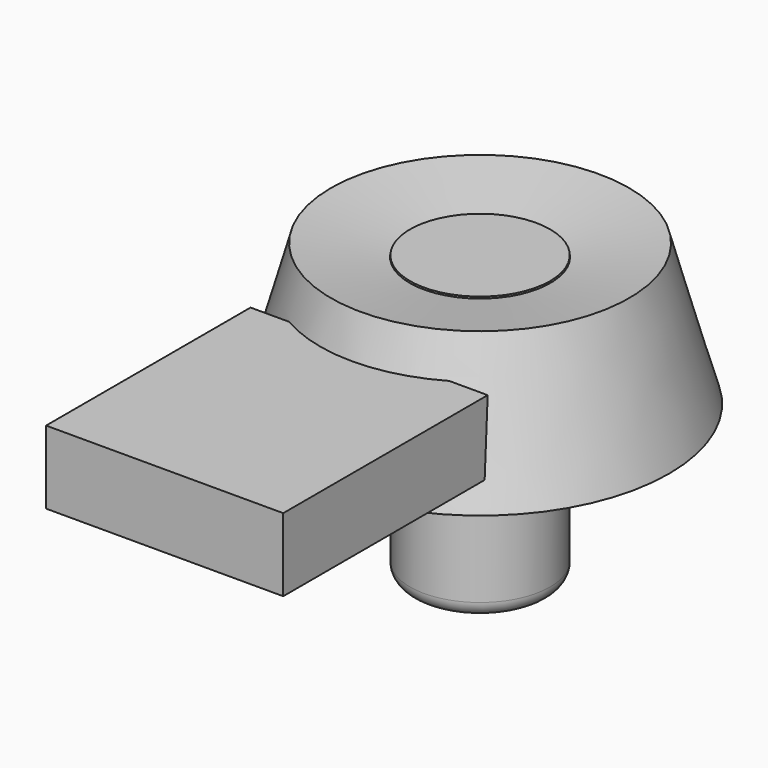
from build123d import *

# Parameters (mm, degrees)
F3_R     = 22.515409418
F4_DEPTH = 45.72
F5_R     = 4.9056819587
F7_DEPTH = 38.1


# Not quite as in the source:
# - a variable given as a bare number and used for a length is read in inches; the dataset says mm whatever the document's units were


with BuildPart() as f2:
    # F1 (on Front) → F2 (revolve)
    with BuildSketch(Plane.XZ):
        Polygon((-22.5897803903, 45.1795645058), (-47.9269698262, 49.1480380297), (-60.7481971383, 3.6632046103), align=None)
    revolve(axis=Axis((0, 0, 28.5424944013), (0, 0, -1)))

    # F6 (on Right) → F7 (join, symmetric)
    with BuildSketch(Plane.YZ):
        Polygon((-45.7901023328, 13.1264971569), (-44.5690304041, 36.6320833564), (-126.6859471798, 36.6320833564), (-126.6859471798, 13.1264971569), align=None)
    extrude(amount=F7_DEPTH, both=True)


with BuildPart() as f4:
    # F3 (on Top) → F4 (new body, symmetric)
    with BuildSketch(Plane.XY):
        Circle(F3_R)
    extrude(amount=F4_DEPTH, both=True)

    # F5
    f5_edges = [f4.edges().sort_by_distance(p)[0] for p in [
        (-22.515409, 0, -45.72),
    ]]
    fillet(f5_edges, radius=F5_R)


solid = Compound([f2.part, f4.part])
